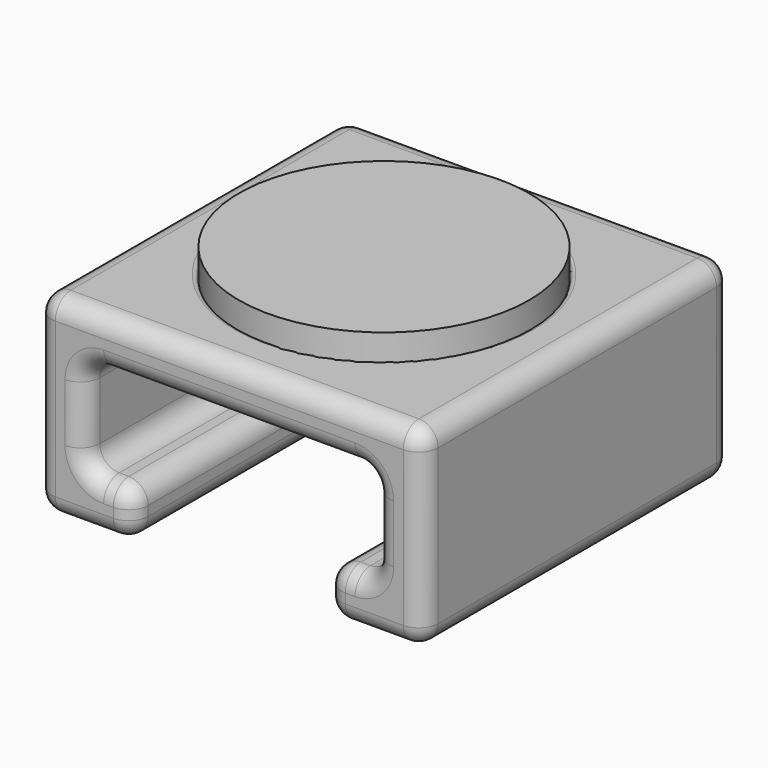
from build123d import *

# Parameters (mm, degrees)
F1_DEPTH = 12.7
F2_R     = 4.7625
F3_DEPTH = 0.79375
F4_F1_R  = 0.635
F4_F2_R  = 0.635
F5_R     = 0.15875
F7_R     = 4.7625
F8_DEPTH = 1.5875


with BuildPart() as f1:
    # F0 (on Front) → F1 (new body)
    with BuildSketch(Plane.XZ):
        Polygon((6.35, 0), (-6.35, 0), (-6.35, -6.35), (-3.175, -6.35), (-3.175, -4.7625), (-4.7625, -4.7625), (-4.7625, -1.5875), (4.7625, -1.5875), (4.7625, -4.7625), (3.175, -4.7625), (3.175, -6.35), (6.35, -6.35), align=None)
    extrude(amount=F1_DEPTH)

    # F2 (on face) → F3 (cut)
    with BuildSketch(Plane.XY):
        with Locations((0, -6.35)):
            Circle(F2_R)
    extrude(amount=-F3_DEPTH, mode=Mode.SUBTRACT)

    # F4: fillet of radius 0.635 on 35 edges, made by hand

    # F4_f1
    f4_f1_edges = [f1.edges().sort_by_distance(p)[0] for p in [
        (-4.7625, -6.35, -4.7625),
        (-4.7625, -6.35, -1.5875),
        (4.7625, -6.35, -1.5875),
        (4.7625, -6.35, -4.7625),
    ]]
    fillet(f4_f1_edges, radius=F4_F1_R)

    # F4_f2
    f4_f2_edges = [f1.edges().sort_by_distance(p)[0] for p in [
        (0, 0, 0),
        (-6.35, -6.35, 0),
        (0, -12.7, 0),
        (6.35, -6.35, 0),
        (-6.35, 0, -3.175),
        (-6.35, -12.7, -3.175),
        (6.35, 0, -3.175),
        (6.35, -12.7, -3.175),
        (-6.35, -6.35, -6.35),
        (-4.7625, 0, -6.35),
        (-3.175, -6.35, -6.35),
        (-4.7625, -12.7, -6.35),
        (-3.175, 0, -5.55625),
        (-3.175, -12.7, -5.55625),
        (-3.65125, 0, -4.7625),
        (-4.7625, 0, -3.175),
        (0, 0, -1.5875),
        (-3.175, -6.35, -4.7625),
        (3.175, 0, -5.55625),
        (3.65125, 0, -4.7625),
        (4.7625, 0, -3.175),
        (4.7625, 0, -6.35),
        (4.7625, -12.7, -3.175),
        (3.175, -6.35, -4.7625),
        (3.175, -6.35, -6.35),
        (6.35, -6.35, -6.35),
        (3.65125, -12.7, -4.7625),
        (4.7625, -12.7, -6.35),
        (3.175, -12.7, -5.55625),
        (-4.7625, -12.7, -3.175),
        (0, -12.7, -1.5875),
        (-4.5765128061, -12.7, -1.7734871939),
        (4.5765128061, -12.7, -1.7734871939),
        (-4.5765128061, -12.7, -4.5765128061),
        (4.5765128061, -12.7, -4.5765128061),
        (4.5765128061, 0, -1.7734871939),
        (4.5765128061, 0, -4.5765128061),
        (-4.5765128061, 0, -1.7734871939),
        (-4.5765128061, 0, -4.5765128061),
    ]]
    fillet(f4_f2_edges, radius=F4_F2_R)

    # F5
    f5_edges = [f1.edges().sort_by_distance(p)[0] for p in [
        (-4.7625, -6.35, 0),
        (-4.7625, -6.35, -0.79375),
    ]]
    fillet(f5_edges, radius=F5_R)


with BuildPart() as f8:
    # F7 (on offset) → F8 (new body)
    with BuildSketch(Plane.XY.offset(-0.79375)):
        with Locations((0, -6.35)):
            Circle(F7_R)
    extrude(amount=F8_DEPTH)


solid = Compound([f1.part, f8.part])
